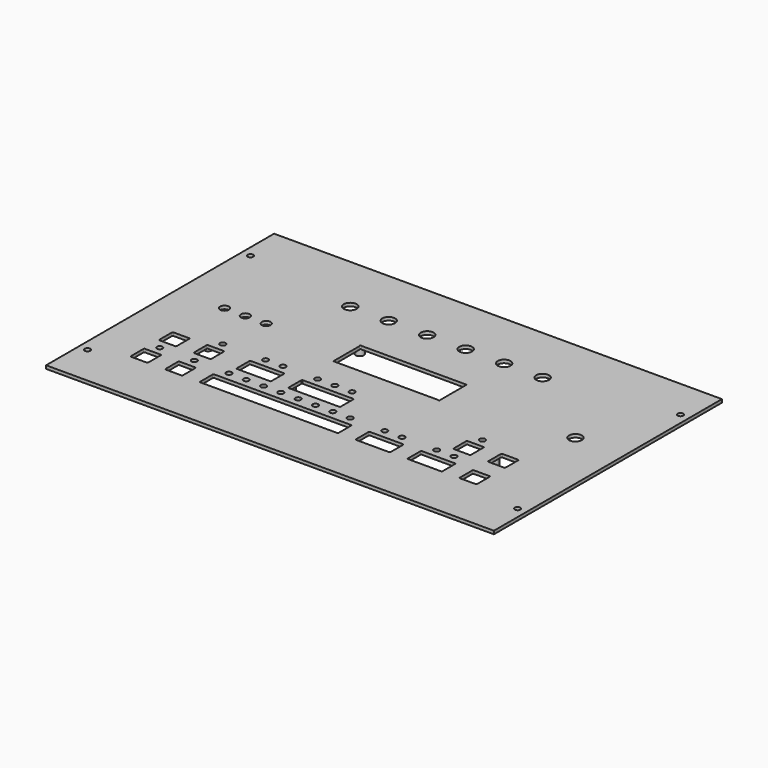
from build123d import *

# Parameters (mm, degrees)
F1_R     = 1.75
F1_R_2   = 2.75
F1_R_3   = 4
F2_DEPTH = 2
F4_R     = 2.5
F5_DEPTH = 6
F6_DEPTH = 5


# Not quite as in the source:
# - ends of sketch curves that miss each other by under 0.0002 mm in the source are joined


with BuildPart() as f2:
    # F1 (on face) → F2 (new body)
    with BuildSketch(Plane.XY):
        Polygon((140.2, -88.4), (140.2, 89.4), (-139.2, 89.4), (-139.2, -88.4), (-138.2, -88.4), align=None)
        with Locations((-133.665, -63)):
            Circle(F1_R, mode=Mode.SUBTRACT)
        with BuildLine():
            ThreePointArc((-112.95, -45.25), (-112.8035533906, -44.8964466094), (-112.45, -44.75))
            Line((-112.45, -44.75), (-102.65, -44.75))
            ThreePointArc((-102.65, -44.75), (-102.2964466094, -44.8964466094), (-102.15, -45.25))
            Line((-102.15, -45.25), (-102.15, -55.05))
            ThreePointArc((-102.15, -55.05), (-102.2964466094, -55.4035533906), (-102.65, -55.55))
            Line((-102.65, -55.55), (-112.45, -55.55))
            ThreePointArc((-112.45, -55.55), (-112.8035533906, -55.4035533906), (-112.95, -55.05))
            Line((-112.95, -55.05), (-112.95, -45.25))
        make_face(mode=Mode.SUBTRACT)
        with BuildLine():
            ThreePointArc((-80.55, -55.05), (-80.6964466094, -55.4035533906), (-81.05, -55.55))
            Line((-81.05, -55.55), (-90.85, -55.55))
            ThreePointArc((-90.85, -55.55), (-91.2035533906, -55.4035533906), (-91.35, -55.05))
            Line((-91.35, -55.05), (-91.35, -45.25))
            ThreePointArc((-91.35, -45.25), (-91.2035533906, -44.8964466094), (-90.85, -44.75))
            Line((-90.85, -44.75), (-81.05, -44.75))
            ThreePointArc((-81.05, -44.75), (-80.6964466094, -44.8964466094), (-80.55, -45.25))
            Line((-80.55, -45.25), (-80.55, -55.05))
        make_face(mode=Mode.SUBTRACT)
        with BuildLine():
            ThreePointArc((-69.25, -55.55), (-69.6035533906, -55.4035533906), (-69.75, -55.05))
            Line((-69.75, -55.05), (-69.75, -45.25))
            ThreePointArc((-69.75, -45.25), (-69.6035533906, -44.8964466094), (-69.25, -44.75))
            Line((-69.25, -44.75), (16.15, -44.75))
            ThreePointArc((16.15, -44.75), (16.5035533906, -44.8964466094), (16.65, -45.25))
            Line((16.65, -45.25), (16.65, -55.05))
            ThreePointArc((16.65, -55.05), (16.5035533906, -55.4035533906), (16.15, -55.55))
            Line((16.15, -55.55), (-69.25, -55.55))
        make_face(mode=Mode.SUBTRACT)
        with Locations((-107.55, -39.35)):
            Circle(F1_R, mode=Mode.SUBTRACT)
        with BuildLine():
            ThreePointArc((-102.65, -22.55), (-102.2964466094, -22.6964466094), (-102.15, -23.05))
            Line((-102.15, -23.05), (-102.15, -32.85))
            ThreePointArc((-102.15, -32.85), (-102.2964466094, -33.2035533906), (-102.65, -33.35))
            Line((-102.65, -33.35), (-112.45, -33.35))
            ThreePointArc((-112.45, -33.35), (-112.8035533906, -33.2035533906), (-112.95, -32.85))
            Line((-112.95, -32.85), (-112.95, -23.05))
            ThreePointArc((-112.95, -23.05), (-112.8035533906, -22.6964466094), (-112.45, -22.55))
            Line((-112.45, -22.55), (-102.65, -22.55))
        make_face(mode=Mode.SUBTRACT)
        with Locations((-85.95, -39.35)):
            Circle(F1_R, mode=Mode.SUBTRACT)
        with BuildLine():
            ThreePointArc((-91.35, -23.05), (-91.2035533906, -22.6964466094), (-90.85, -22.55))
            Line((-90.85, -22.55), (-81.05, -22.55))
            ThreePointArc((-81.05, -22.55), (-80.6964466094, -22.6964466094), (-80.55, -23.05))
            Line((-80.55, -23.05), (-80.55, -32.85))
            ThreePointArc((-80.55, -32.85), (-80.6964466094, -33.2035533906), (-81.05, -33.35))
            Line((-81.05, -33.35), (-90.85, -33.35))
            ThreePointArc((-90.85, -33.35), (-91.2035533906, -33.2035533906), (-91.35, -32.85))
            Line((-91.35, -32.85), (-91.35, -23.05))
        make_face(mode=Mode.SUBTRACT)
        with Locations((-85.95, -17.15)):
            Circle(F1_R, mode=Mode.SUBTRACT)
        with Locations((-64.35, -39.35)):
            Circle(F1_R, mode=Mode.SUBTRACT)
        with Locations((-53.55, -39.35)):
            Circle(F1_R, mode=Mode.SUBTRACT)
        with Locations((-42.75, -39.35)):
            Circle(F1_R, mode=Mode.SUBTRACT)
        with BuildLine():
            ThreePointArc((-64.65, -23.05), (-64.5035533906, -22.6964466094), (-64.15, -22.55))
            Line((-64.15, -22.55), (-43.55, -22.55))
            ThreePointArc((-43.55, -22.55), (-43.1964466094, -22.6964466094), (-43.05, -23.05))
            Line((-43.05, -23.05), (-43.05, -32.85))
            ThreePointArc((-43.05, -32.85), (-43.1964466094, -33.2035533906), (-43.55, -33.35))
            Line((-43.55, -33.35), (-64.15, -33.35))
            ThreePointArc((-64.15, -33.35), (-64.5035533906, -33.2035533906), (-64.65, -32.85))
            Line((-64.65, -32.85), (-64.65, -23.05))
        make_face(mode=Mode.SUBTRACT)
        with Locations((-31.95, -39.35)):
            Circle(F1_R, mode=Mode.SUBTRACT)
        with Locations((-21.15, -39.35)):
            Circle(F1_R, mode=Mode.SUBTRACT)
        with Locations((-10.35, -39.35)):
            Circle(F1_R, mode=Mode.SUBTRACT)
        with Locations((0.45, -39.35)):
            Circle(F1_R, mode=Mode.SUBTRACT)
        with BuildLine():
            ThreePointArc((-32.25, -23.05), (-32.1035533906, -22.6964466094), (-31.75, -22.55))
            Line((-31.75, -22.55), (-0.35, -22.55))
            ThreePointArc((-0.35, -22.55), (0.0035533906, -22.6964466094), (0.15, -23.05))
            Line((0.15, -23.05), (0.15, -32.85))
            ThreePointArc((0.15, -32.85), (0.0035533906, -33.2035533906), (-0.35, -33.35))
            Line((-0.35, -33.35), (-31.75, -33.35))
            ThreePointArc((-31.75, -33.35), (-32.1035533906, -33.2035533906), (-32.25, -32.85))
            Line((-32.25, -32.85), (-32.25, -23.05))
        make_face(mode=Mode.SUBTRACT)
        with Locations((-59.25, -17.15)):
            Circle(F1_R, mode=Mode.SUBTRACT)
        with Locations((-48.45, -17.15)):
            Circle(F1_R, mode=Mode.SUBTRACT)
        with Locations((-26.85, -17.15)):
            Circle(F1_R, mode=Mode.SUBTRACT)
        with Locations((-16.05, -17.15)):
            Circle(F1_R, mode=Mode.SUBTRACT)
        with Locations((-5.25, -17.15)):
            Circle(F1_R, mode=Mode.SUBTRACT)
        with BuildLine():
            ThreePointArc((27.95, -55.55), (27.5964466094, -55.4035533906), (27.45, -55.05))
            Line((27.45, -55.05), (27.45, -45.25))
            ThreePointArc((27.45, -45.25), (27.5964466094, -44.8964466094), (27.95, -44.75))
            Line((27.95, -44.75), (48.55, -44.75))
            ThreePointArc((48.55, -44.75), (48.9035533906, -44.8964466094), (49.05, -45.25))
            Line((49.05, -45.25), (49.05, -55.05))
            ThreePointArc((49.05, -55.05), (48.9035533906, -55.4035533906), (48.55, -55.55))
            Line((48.55, -55.55), (27.95, -55.55))
        make_face(mode=Mode.SUBTRACT)
        with BuildLine():
            ThreePointArc((59.85, -45.25), (59.9964466094, -44.8964466094), (60.35, -44.75))
            Line((60.35, -44.75), (80.95, -44.75))
            ThreePointArc((80.95, -44.75), (81.3035533906, -44.8964466094), (81.45, -45.25))
            Line((81.45, -45.25), (81.45, -55.05))
            ThreePointArc((81.45, -55.05), (81.3035533906, -55.4035533906), (80.95, -55.55))
            Line((80.95, -55.55), (60.35, -55.55))
            ThreePointArc((60.35, -55.55), (59.9964466094, -55.4035533906), (59.85, -55.05))
            Line((59.85, -55.05), (59.85, -45.25))
        make_face(mode=Mode.SUBTRACT)
        with BuildLine():
            ThreePointArc((102.55, -44.75), (102.9035533906, -44.8964466094), (103.05, -45.25))
            Line((103.05, -45.25), (103.05, -55.05))
            ThreePointArc((103.05, -55.05), (102.9035533906, -55.4035533906), (102.55, -55.55))
            Line((102.55, -55.55), (92.75, -55.55))
            ThreePointArc((92.75, -55.55), (92.3964466094, -55.4035533906), (92.25, -55.05))
            Line((92.25, -55.05), (92.25, -45.25))
            ThreePointArc((92.25, -45.25), (92.3964466094, -44.8964466094), (92.75, -44.75))
            Line((92.75, -44.75), (102.55, -44.75))
        make_face(mode=Mode.SUBTRACT)
        with Locations((134.665, -63)):
            Circle(F1_R, mode=Mode.SUBTRACT)
        with Locations((11.25, -39.35)):
            Circle(F1_R, mode=Mode.SUBTRACT)
        with Locations((32.85, -39.35)):
            Circle(F1_R, mode=Mode.SUBTRACT)
        with Locations((43.65, -39.35)):
            Circle(F1_R, mode=Mode.SUBTRACT)
        with Locations((65.25, -39.35)):
            Circle(F1_R, mode=Mode.SUBTRACT)
        with Locations((76.05, -39.35)):
            Circle(F1_R, mode=Mode.SUBTRACT)
        with BuildLine():
            ThreePointArc((71.15, -33.35), (70.7964466094, -33.2035533906), (70.65, -32.85))
            Line((70.65, -32.85), (70.65, -23.05))
            ThreePointArc((70.65, -23.05), (70.7964466094, -22.6964466094), (71.15, -22.55))
            Line((71.15, -22.55), (80.95, -22.55))
            ThreePointArc((80.95, -22.55), (81.3035533906, -22.6964466094), (81.45, -23.05))
            Line((81.45, -23.05), (81.45, -32.85))
            ThreePointArc((81.45, -32.85), (81.3035533906, -33.2035533906), (80.95, -33.35))
            Line((80.95, -33.35), (71.15, -33.35))
        make_face(mode=Mode.SUBTRACT)
        with BuildLine():
            ThreePointArc((103.05, -32.85), (102.9035533906, -33.2035533906), (102.55, -33.35))
            Line((102.55, -33.35), (92.75, -33.35))
            ThreePointArc((92.75, -33.35), (92.3964466094, -33.2035533906), (92.25, -32.85))
            Line((92.25, -32.85), (92.25, -23.05))
            ThreePointArc((92.25, -23.05), (92.3964466094, -22.6964466094), (92.75, -22.55))
            Line((92.75, -22.55), (102.55, -22.55))
            ThreePointArc((102.55, -22.55), (102.9035533906, -22.6964466094), (103.05, -23.05))
            Line((103.05, -23.05), (103.05, -32.85))
        make_face(mode=Mode.SUBTRACT)
        with Locations((76.05, -17.15)):
            Circle(F1_R, mode=Mode.SUBTRACT)
        with Locations((-108.95, 12.96)):
            Circle(F1_R_2, mode=Mode.SUBTRACT)
        with Locations((-95.95, 12.96)):
            Circle(F1_R_2, mode=Mode.SUBTRACT)
        with Locations((-82.95, 12.96)):
            Circle(F1_R_2, mode=Mode.SUBTRACT)
        with Locations((-133.665, 64)):
            Circle(F1_R, mode=Mode.SUBTRACT)
        with Locations((-62.2, 52.55)):
            Circle(F1_R_3, mode=Mode.SUBTRACT)
        with Locations((-38.2, 52.55)):
            Circle(F1_R_3, mode=Mode.SUBTRACT)
        with Locations((-14.2, 52.55)):
            Circle(F1_R_3, mode=Mode.SUBTRACT)
        with BuildLine():
            ThreePointArc((-32.5999936284, 22.8530063581), (-32.5935533906, 23.5535533906), (-31.8930063581, 23.5599936284))
            Line((-31.8930063581, 23.5599936284), (32.893, 23.56))
            ThreePointArc((32.893, 23.56), (33.5935533906, 23.5535533906), (33.5999936284, 22.8530063581))
            Line((33.5999936284, 22.8530063581), (33.6, 3.067))
            ThreePointArc((33.6, 3.067), (33.5935533906, 2.3664466094), (32.8930063581, 2.3600063716))
            Line((32.8930063581, 2.3600063716), (-31.893, 2.36))
            ThreePointArc((-31.893, 2.36), (-32.5935533906, 2.3664466094), (-32.5999936284, 3.0669936419))
            Line((-32.5999936284, 3.0669936419), (-32.5999936284, 22.8530063581))
        make_face(mode=Mode.SUBTRACT)
        with Locations((109.95, 12.96)):
            Circle(F1_R_3, mode=Mode.SUBTRACT)
        with Locations((9.8, 52.55)):
            Circle(F1_R_3, mode=Mode.SUBTRACT)
        with Locations((33.8, 52.55)):
            Circle(F1_R_3, mode=Mode.SUBTRACT)
        with Locations((57.8, 52.55)):
            Circle(F1_R_3, mode=Mode.SUBTRACT)
        with Locations((134.665, 64)):
            Circle(F1_R, mode=Mode.SUBTRACT)
    extrude(amount=F2_DEPTH)

    # F4 (on face) → F5 (join)
    with BuildSketch(Plane(origin=(0, 0, 0), x_dir=(1, 0, 0), z_dir=(0, 0, -1))):
        with Locations((-37, -28.46)):
            Circle(F4_R)
        with Locations((-37, 2.54)):
            Circle(F4_R)
        with Locations((38, 2.54)):
            Circle(F4_R)
        with Locations((38, -28.46)):
            Circle(F4_R)
    extrude(amount=F5_DEPTH)

    # F4 (on face) → F6 (join)
    with BuildSketch(Plane(origin=(0, 0, 0), x_dir=(1, 0, 0), z_dir=(0, 0, -1))):
        with Locations((45.8, -52.55)):
            Circle(F4_R)
        with Locations((109.05, -33.65)):
            Circle(F4_R)
        with Locations((110.85, -23.05)):
            Circle(F4_R)
        with Locations((107.6, 3.75)):
            Circle(F4_R)
        with Locations((88.35, 23.15)):
            Circle(F4_R)
        with Locations((110.35, 50.15)):
            Circle(F4_R)
        with Locations((21.35, 50.15)):
            Circle(F4_R)
        with Locations((5.35, 17.15)):
            Circle(F4_R)
        with Locations((-38.65, 23.15)):
            Circle(F4_R)
        with Locations((-96.65, 15.15)):
            Circle(F4_R)
        with Locations((-96.65, 50.15)):
            Circle(F4_R)
        with Locations((-89.45, -6.55)):
            Circle(F4_R)
        with Locations((-89.45, -33.55)):
            Circle(F4_R)
        with Locations((-45.05, -34.65)):
            Circle(F4_R)
        with Locations((-50.2, -52.55)):
            Circle(F4_R)
        with Locations((-2.2, -52.55)):
            Circle(F4_R)
    extrude(amount=F6_DEPTH)


solid = f2.part
